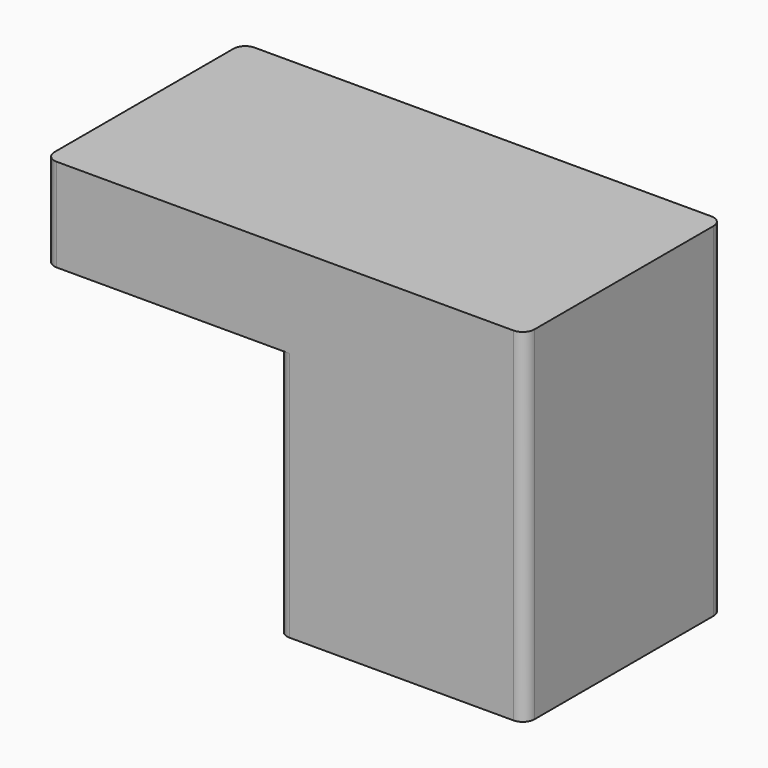
from build123d import *

# Parameters (mm, degrees)
F0_W      = 42.5
F0_H      = 42.5
F0_W_2    = 38.5
F0_H_2    = 38.5
F1_DEPTH  = 20
F3_DEPTH  = 38
F4_W      = 42.5
F4_H      = 42.5
F5_DEPTH  = 1
F9_DEPTH  = 2.5
F11_DEPTH = 38
F12_W     = 42.5
F12_H     = 16
F13_DEPTH = 2
F15_DEPTH = 38
F16_R     = 1.99999


# Not quite as in the source:
# - a fillet or chamfer is up to 0.001 mm smaller than in the source, because OpenCascade refuses the exact size


with BuildPart() as f1:
    # F0 (on Top) → F1 (new body)
    with BuildSketch(Plane.XY):
        Rectangle(F0_W, F0_H)
        Rectangle(F0_W_2, F0_H_2, mode=Mode.SUBTRACT)
    extrude(amount=-F1_DEPTH)

    # F2 (on face) → F3 (join)
    with BuildSketch(Plane.XY):
        Polygon((-21.25, -19.25), (-21.25, -21.25), (21.25, -21.25), (21.25, 21.25), (-21.25, 21.25), (-21.25, 19.25), (-19.25, 19.25), (19.25, 19.25), (19.25, -19.25), (-19.25, -19.25), align=None)
    extrude(amount=F3_DEPTH)

    # F4 (on face) → F5 (join)
    with BuildSketch(Plane.XY.offset(38)):
        Rectangle(F4_W, F4_H)
    extrude(amount=F5_DEPTH)

    # F8 (on plane+point) → F9 (join, symmetric)
    with BuildSketch(Plane(origin=(0, 0, 0), x_dir=(-1, 0, 0), z_dir=(0, 1, 0))):
        with BuildLine():
            Line((21.25, 37.7357607819), (21.25, 38))
            Line((21.25, 38), (-19.25, 38))
            Line((-19.25, 38), (-19.25, 0))
            Line((-19.25, 0), (-17.25, 0))
            Line((-17.25, 0), (-17.25, 10.2847843622))
            ThreePointArc((-17.25, 10.2847843622), (-13.3594316189, 22.1374723659), (-3.2013787085, 29.3787910519))
            Line((-3.2013787085, 29.3787910519), (20.5475689354, 36.7810604474))
            ThreePointArc((20.5475689354, 36.7810604474), (21.0554715809, 37.1431263817), (21.25, 37.7357607819))
        make_face()
    extrude(amount=F9_DEPTH, both=True)

    # F10 (on face) → F11 (join)
    with BuildSketch(Plane(origin=(-21.25, 0, 0), x_dir=(0, -1, 0), z_dir=(-1, 0, 0))):
        Polygon((2.5, 38), (19.25, 38), (19.25, 23), (21.25, 23), (21.25, 39), (-21.25, 39), (-21.25, 23), (-19.25, 23), (-19.25, 38), (-2.5, 38), align=None)
    extrude(amount=F11_DEPTH)

    # F12 (on face) → F13 (join)
    with BuildSketch(Plane(origin=(-59.25, 0, 0), x_dir=(0, -1, 0), z_dir=(-1, 0, 0))):
        with Locations((0, 31)):
            Rectangle(F12_W, F12_H)
    extrude(amount=F13_DEPTH)

    # F14 (on face) → F15 (join, through all)
    with BuildSketch(Plane(origin=(0, 0, 38), x_dir=(1, 0, 0), z_dir=(0, 0, -1))):
        with BuildLine():
            Line((2.5, 18.25), (2.5, 19.25))
            Line((2.5, 19.25), (-2.5, 19.25))
            Line((-2.5, 19.25), (-2.5, 18.25))
            ThreePointArc((-2.5, 18.25), (-2.2071067812, 17.5428932188), (-1.5, 17.25))
            Line((-1.5, 17.25), (1.5, 17.25))
            ThreePointArc((1.5, 17.25), (2.2071067812, 17.5428932188), (2.5, 18.25))
        make_face()
        with BuildLine():
            Line((-2.5, -18.25), (-2.5, -19.25))
            Line((-2.5, -19.25), (2.5, -19.25))
            Line((2.5, -19.25), (2.5, -18.25))
            ThreePointArc((2.5, -18.25), (2.2071067812, -17.5428932188), (1.5, -17.25))
            Line((1.5, -17.25), (-1.5, -17.25))
            ThreePointArc((-1.5, -17.25), (-2.2071067812, -17.5428932188), (-2.5, -18.25))
        make_face()
    extrude(amount=F15_DEPTH)

    # F16 (radius 2 in the source; OpenCascade refuses exactly that, so slightly less here)
    f16_edges = [f1.edges().sort_by_distance(p)[0] for p in [
        (21.25, 21.25, 9.5),
        (-21.25, 21.25, 1.5),
        (-61.25, 21.25, 31),
        (-61.25, -21.25, 31),
        (-21.25, -21.25, 1.5),
        (21.25, -21.25, 9.5),
    ]]
    fillet(f16_edges, radius=F16_R)


solid = f1.part
